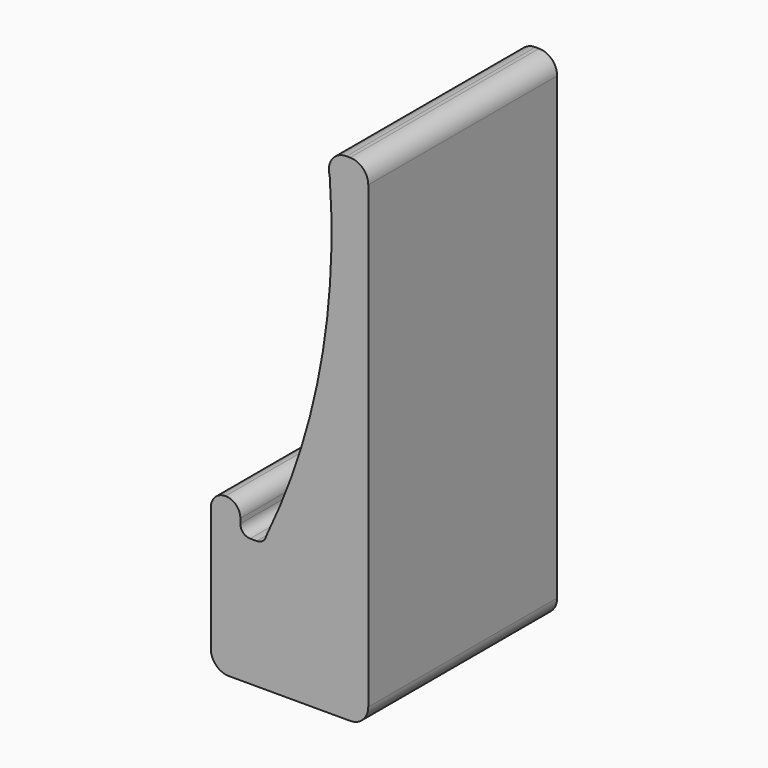
from build123d import *

# Parameters (mm, degrees)
F1_DEPTH = 76.2


# Not quite as in the source:
# - ends of sketch curves that miss each other by under 0.0002 mm in the source are joined


with BuildPart() as f1:
    # F0 (on Front) → F1 (new body)
    with BuildSketch(Plane.XZ):
        with BuildLine():
            Line((-25.4, -33.9672422), (-25.4, -74.1627422))
            ThreePointArc((-25.4, -74.1627422), (-23.6889178157, -78.2936600157), (-19.558, -80.0047422))
            Line((-19.558, -80.0047422), (19.558, -80.0047422))
            ThreePointArc((19.558, -80.0047422), (23.6889178157, -78.2936600157), (25.4, -74.1627422))
            Line((25.4, -74.1627422), (25.4, 74.1618532))
            ThreePointArc((25.4, 74.1618532), (23.6889178157, 78.2927710157), (19.558, 80.0038532))
            Line((19.558, 80.0038532), (18.3634634, 80.0038532))
            ThreePointArc((18.3634634, 80.0038532), (13.9275587532, 77.9297664461), (12.844644278, 73.1541629443))
            ThreePointArc((12.844644278, 73.1541629443), (12.9337447112, 72.6965968013), (12.9860822326, 72.2333837478))
            ThreePointArc((12.9860822326, 72.2333837478), (9.8726352632, 17.0060097148), (-7.2204417887, -35.601816093))
            ThreePointArc((-7.2204417887, -35.601816093), (-7.3997485398, -36.0211585586), (-7.5457824697, -36.4532160254))
            ThreePointArc((-7.5457824697, -36.4532160254), (-8.6899630694, -38.0977002575), (-10.5910126, -38.7297422))
            Line((-10.5910126, -38.7297422), (-12.7, -38.7297422))
            ThreePointArc((-12.7, -38.7297422), (-14.9450640303, -37.7998062303), (-15.875, -35.5547422))
            Line((-15.875, -35.5547422), (-15.875, -33.9672422))
            ThreePointArc((-15.875, -33.9672422), (-17.2699039546, -30.5996461546), (-20.6375, -29.2047422))
            ThreePointArc((-20.6375, -29.2047422), (-24.0050960454, -30.5996461546), (-25.4, -33.9672422))
        make_face()
    extrude(amount=F1_DEPTH)


solid = f1.part
